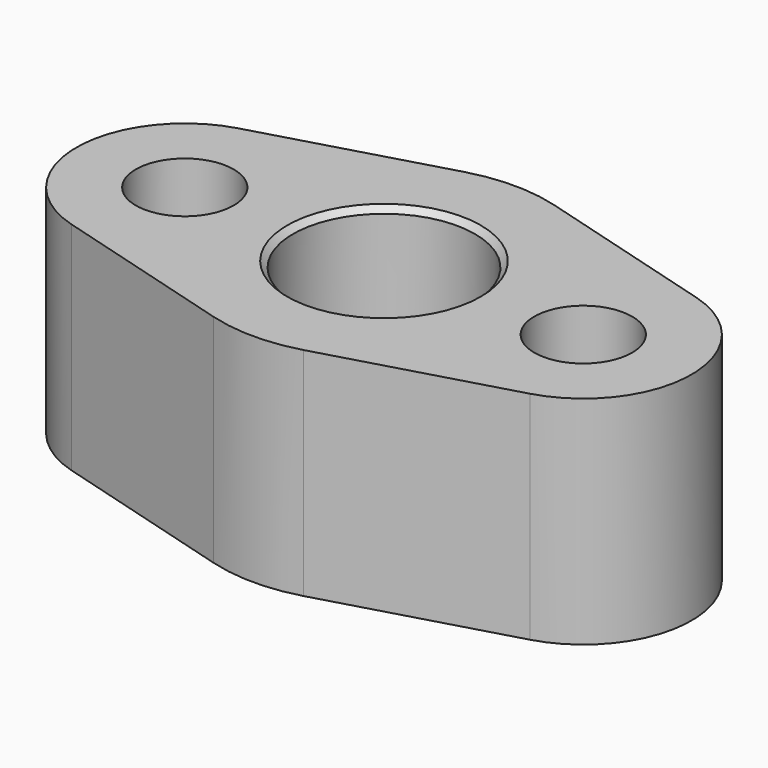
from build123d import *

# Parameters (mm, degrees)
F0_R     = 2.15265
F0_R_2   = 4
F1_DEPTH = 7.9375
F2_SIZE  = 0.254
F3_R     = 2.15265
F3_R_2   = 4
F3_R_3   = 2.4125
F4_DEPTH = 1.5875


with BuildPart() as f1:
    # F0 (on Top) → F1 (new body)
    with BuildSketch(Plane.XY):
        with BuildLine():
            Line((10.0737161198, 4.5784406229), (1.9754279601, 6.8977031956))
            ThreePointArc((1.9754279601, 6.8977031956), (0, 7.175), (-1.9754279601, 6.8977031956))
            Line((-1.9754279601, 6.8977031956), (-10.0737161198, 4.5784406229))
            ThreePointArc((-10.0737161198, 4.5784406229), (-13.525, 0), (-10.0737161198, -4.5784406229))
            Line((-10.0737161198, -4.5784406229), (-1.9754279601, -6.8977031956))
            ThreePointArc((-1.9754279601, -6.8977031956), (0, -7.175), (1.9754279601, -6.8977031956))
            Line((1.9754279601, -6.8977031956), (10.0737161198, -4.5784406229))
            ThreePointArc((10.0737161198, -4.5784406229), (13.525, 0), (10.0737161198, 4.5784406229))
        make_face()
        with Locations((-8.7625, 0)):
            Circle(F0_R, mode=Mode.SUBTRACT)
        Circle(F0_R_2, mode=Mode.SUBTRACT)
        with Locations((8.7625, 0)):
            Circle(F0_R, mode=Mode.SUBTRACT)
    extrude(amount=F1_DEPTH)

    # F2
    f2_edges = [f1.edges().sort_by_distance(p)[0] for p in [
        (-4, 0, 7.9375),
    ]]
    chamfer(f2_edges, length=F2_SIZE)

    # F3 (on face) → F4 (join)
    with BuildSketch(Plane(origin=(0, 0, 0), x_dir=(1, 0, 0), z_dir=(0, 0, -1))):
        with BuildLine():
            ThreePointArc((10.0737161198, -4.5784406229), (13.525, 0), (10.0737161198, 4.5784406229))
            Line((10.0737161198, 4.5784406229), (1.9754279601, 6.8977031956))
            ThreePointArc((1.9754279601, 6.8977031956), (0, 7.175), (-1.9754279601, 6.8977031956))
            Line((-1.9754279601, 6.8977031956), (-10.0737161198, 4.5784406229))
            ThreePointArc((-10.0737161198, 4.5784406229), (-13.525, 0), (-10.0737161198, -4.5784406229))
            Line((-10.0737161198, -4.5784406229), (-1.9754279601, -6.8977031956))
            ThreePointArc((-1.9754279601, -6.8977031956), (0, -7.175), (1.9754279601, -6.8977031956))
            Line((1.9754279601, -6.8977031956), (10.0737161198, -4.5784406229))
        make_face()
        with Locations((-8.7625, 0)):
            Circle(F3_R, mode=Mode.SUBTRACT)
        Circle(F3_R_2, mode=Mode.SUBTRACT)
        with Locations((8.7625, 0)):
            Circle(F3_R, mode=Mode.SUBTRACT)
        Circle(F3_R_2)
        Circle(F3_R_3, mode=Mode.SUBTRACT)
    extrude(amount=F4_DEPTH)


solid = f1.part
